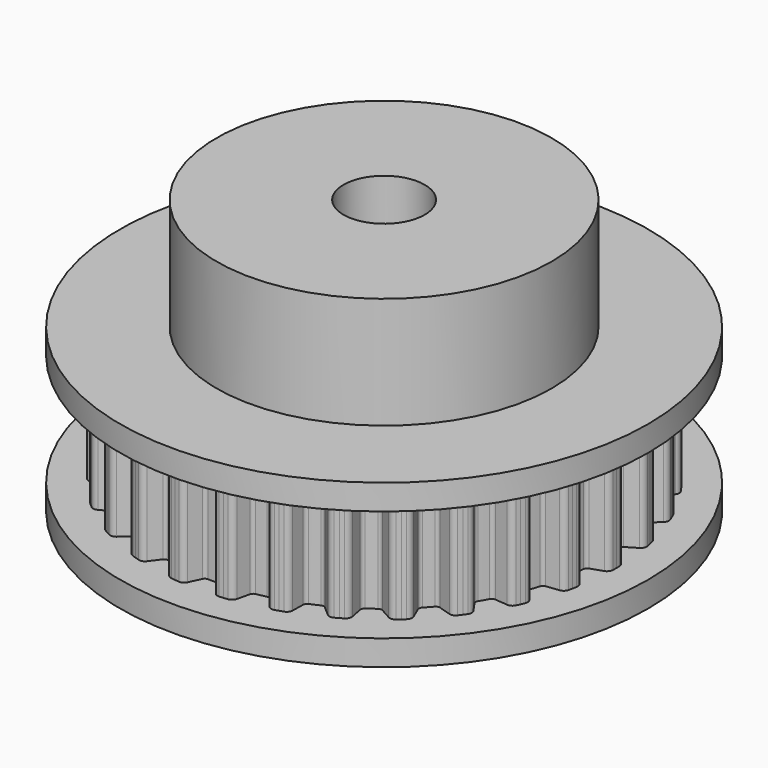
from build123d import *

# Parameters (mm, degrees)
F3_DEPTH  = 5.5
F4_COUNT  = 30
F5_R      = 26
F6_DEPTH  = 2.5
F7_R      = 26
F8_DEPTH  = 2.5
F9_R      = 16.5
F10_DEPTH = 11
F11_R     = 4
F12_DEPTH = 27.001


# Not quite as in the source:
# - a feature names something its author has since deleted; it is built from what else it names


with BuildPart() as f3:
    # F2 (on Top) → F3 (new body, symmetric)
    with BuildSketch(Plane.XY):
        with BuildLine():
            Line((0, 0), (2.3909047802, 22.7479394538))
            ThreePointArc((2.3909047802, 22.7479394538), (2.1907733755, 22.7680848355), (1.9904725562, 22.7864695393))
            ThreePointArc((1.9904725562, 22.7864695393), (1.6382245164, 22.7083407848), (1.3944747538, 22.4423166562))
            Line((1.3944747538, 22.4423166562), (0.8610605415, 21.2984061865))
            ThreePointArc((0.8610605415, 21.2984061865), (0.7095263728, 21.1276246157), (0.4892507538, 21.0675613086))
            ThreePointArc((0.4892507538, 21.0675613086), (0, 21.0732414638), (-0.4892507538, 21.0675613086))
            ThreePointArc((-0.4892507538, 21.0675613086), (-0.7095263728, 21.1276246157), (-0.8610605415, 21.2984061865))
            Line((-0.8610605415, 21.2984061865), (-1.3944747538, 22.4423166562))
            ThreePointArc((-1.3944747538, 22.4423166562), (-1.6382245164, 22.7083407848), (-1.9904725562, 22.7864695393))
            ThreePointArc((-1.9904725562, 22.7864695393), (-2.1907733755, 22.7680848355), (-2.3909047802, 22.7479394538))
            Line((-2.3909047802, 22.7479394538), (0, 0))
        make_face()
    extrude(amount=F3_DEPTH, both=True)

    # F4: F3 ×30 about axis
    f4_axis = Axis((0, 0, 0), (0, 0, -1))


with BuildPart() as f3_1:
    add(f3.part)
    for i in range(1, F4_COUNT):
        add(f3.part.rotate(f4_axis, i * 360 / F4_COUNT))

    # F5 (on face) → F6 (join)
    with BuildSketch(Plane.XY.offset(5.5)):
        Circle(F5_R)
    extrude(amount=F6_DEPTH)

    # F7 (on face) → F8 (join)
    with BuildSketch(Plane(origin=(0, 0, -5.5), x_dir=(1, 0, 0), z_dir=(0, 0, -1))):
        Circle(F7_R)
    extrude(amount=F8_DEPTH)

    # F9 (on face) → F10 (join)
    with BuildSketch(Plane.XY.offset(8)):
        Circle(F9_R)
    extrude(amount=F10_DEPTH)

    # F11 (on face) → F12 (cut, through all)
    with BuildSketch(Plane.XY.offset(19)):
        Circle(F11_R)
    extrude(amount=-F12_DEPTH, mode=Mode.SUBTRACT)


solid = f3_1.part
